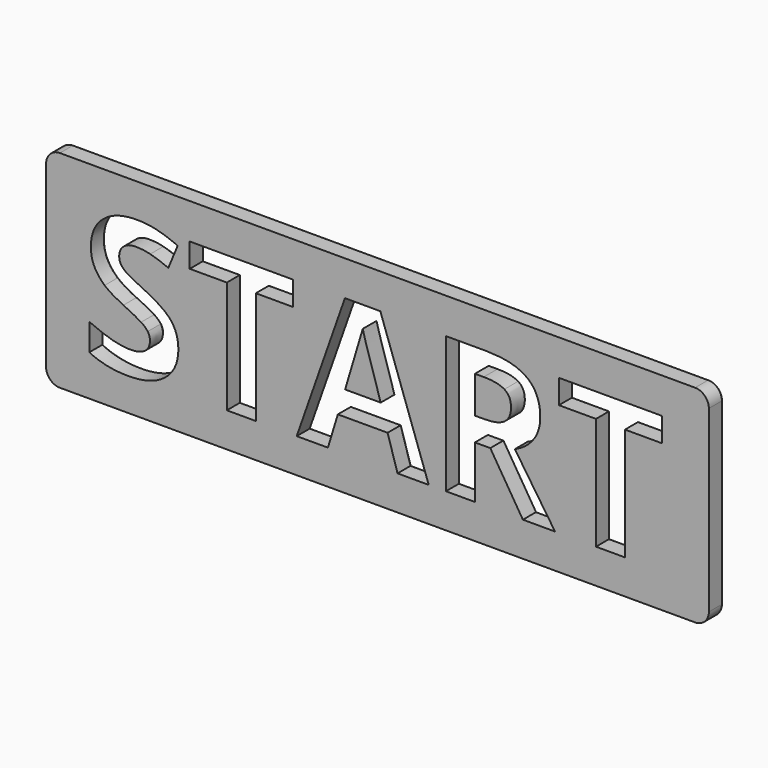
from build123d import *

# Parameters (mm, degrees)
F0_W     = 122.1989149306
F0_H     = 38.1
F1_DEPTH = 3.175
F2_R     = 2.54
F3_R     = 0.254


with BuildPart() as f1:
    # F0 (on Front) → F1 (new body)
    with BuildSketch(Plane.XZ):
        with Locations((54.7494574653, 12.7)):
            Rectangle(F0_W, F0_H)
        with BuildLine():
            add(Edge.make_bspline(
                [(16.7266276042, 11.1538411458), (18.0357638889, 9.4588541667), (18.0357638889, 6.994921875)],
                knots=[0, 0, 0, 1, 1, 1], degree=2))
            add(Edge.make_bspline(
                [(18.0357638889, 6.994921875), (18.0357638889, 3.5828993056), (15.5800998264, 1.6178168403)],
                knots=[0, 0, 0, 1, 1, 1], degree=2))
            add(Edge.make_bspline(
                [(15.5800998264, 1.6178168403), (13.1244357639, -0.347265625), (8.7532986111, -0.347265625)],
                knots=[0, 0, 0, 1, 1, 1], degree=2))
            add(Edge.make_bspline(
                [(8.7532986111, -0.347265625), (4.7184027778, -0.347265625), (1.6205729167, 1.1740885417)],
                knots=[0, 0, 0, 1, 1, 1], degree=2))
            Line((1.6205729167, 1.1740885417), (1.6205729167, 6.1350260417))
            add(Edge.make_bspline(
                [(1.6205729167, 6.1350260417), (4.1671875, 4.9940104167), (5.9338324653, 4.5309895833)],
                knots=[0, 0, 0, 1, 1, 1], degree=2))
            add(Edge.make_bspline(
                [(5.9338324653, 4.5309895833), (7.7004774306, 4.06796875), (9.1667100694, 4.06796875)],
                knots=[0, 0, 0, 1, 1, 1], degree=2))
            add(Edge.make_bspline(
                [(9.1667100694, 4.06796875), (10.9195746528, 4.06796875), (11.8593967014, 4.7376953125)],
                knots=[0, 0, 0, 1, 1, 1], degree=2))
            add(Edge.make_bspline(
                [(11.8593967014, 4.7376953125), (12.79921875, 5.407421875), (12.79921875, 6.7358506944)],
                knots=[0, 0, 0, 1, 1, 1], degree=2))
            add(Edge.make_bspline(
                [(12.79921875, 6.7358506944), (12.79921875, 7.4744791667), (12.3858072917, 8.0532552083)],
                knots=[0, 0, 0, 1, 1, 1], degree=2))
            add(Edge.make_bspline(
                [(12.3858072917, 8.0532552083), (11.9723958333, 8.63203125), (11.1703776042, 9.1639539931)],
                knots=[0, 0, 0, 1, 1, 1], degree=2))
            add(Edge.make_bspline(
                [(11.1703776042, 9.1639539931), (10.368359375, 9.6958767361), (7.9044270833, 10.8699652778)],
                knots=[0, 0, 0, 1, 1, 1], degree=2))
            add(Edge.make_bspline(
                [(7.9044270833, 10.8699652778), (5.6003472222, 11.955859375), (4.4455512153, 12.9535590278)],
                knots=[0, 0, 0, 1, 1, 1], degree=2))
            add(Edge.make_bspline(
                [(4.4455512153, 12.9535590278), (3.2907552083, 13.9512586806), (2.6017361111, 15.2796875)],
                knots=[0, 0, 0, 1, 1, 1], degree=2))
            add(Edge.make_bspline(
                [(2.6017361111, 15.2796875), (1.9127170139, 16.6081163194), (1.9127170139, 18.3775173611)],
                knots=[0, 0, 0, 1, 1, 1], degree=2))
            add(Edge.make_bspline(
                [(1.9127170139, 18.3775173611), (1.9127170139, 21.7233940972), (4.1782118056, 23.6333550347)],
                knots=[0, 0, 0, 1, 1, 1], degree=2))
            add(Edge.make_bspline(
                [(4.1782118056, 23.6333550347), (6.4437065972, 25.5433159722), (10.4400173611, 25.5433159722)],
                knots=[0, 0, 0, 1, 1, 1], degree=2))
            add(Edge.make_bspline(
                [(10.4400173611, 25.5433159722), (12.40234375, 25.5433159722), (14.1855251736, 25.0802951389)],
                knots=[0, 0, 0, 1, 1, 1], degree=2))
            add(Edge.make_bspline(
                [(14.1855251736, 25.0802951389), (15.9687065972, 24.6172743056), (17.9144965278, 23.7739149306)],
                knots=[0, 0, 0, 1, 1, 1], degree=2))
            Line((17.9144965278, 23.7739149306), (16.1947048611, 19.6177517361))
            add(Edge.make_bspline(
                [(16.1947048611, 19.6177517361), (14.1772569444, 20.4445746528), (12.8598524306, 20.7725477431)],
                knots=[0, 0, 0, 1, 1, 1], degree=2))
            add(Edge.make_bspline(
                [(12.8598524306, 20.7725477431), (11.5424479167, 21.1005208333), (10.269140625, 21.1005208333)],
                knots=[0, 0, 0, 1, 1, 1], degree=2))
            add(Edge.make_bspline(
                [(10.269140625, 21.1005208333), (8.7532986111, 21.1005208333), (7.9430121528, 20.3949652778)],
                knots=[0, 0, 0, 1, 1, 1], degree=2))
            add(Edge.make_bspline(
                [(7.9430121528, 20.3949652778), (7.1327256944, 19.6894097222), (7.1327256944, 18.55390625)],
                knots=[0, 0, 0, 1, 1, 1], degree=2))
            add(Edge.make_bspline(
                [(7.1327256944, 18.55390625), (7.1327256944, 17.8483506944), (7.4606987847, 17.3219401042)],
                knots=[0, 0, 0, 1, 1, 1], degree=2))
            add(Edge.make_bspline(
                [(7.4606987847, 17.3219401042), (7.788671875, 16.7955295139), (8.5024956597, 16.3049479167)],
                knots=[0, 0, 0, 1, 1, 1], degree=2))
            add(Edge.make_bspline(
                [(8.5024956597, 16.3049479167), (9.2163194444, 15.8143663194), (11.8842013889, 14.5410590278)],
                knots=[0, 0, 0, 1, 1, 1], degree=2))
            add(Edge.make_bspline(
                [(11.8842013889, 14.5410590278), (15.4174913194, 12.848828125), (16.7266276042, 11.1538411458)],
                knots=[0, 0, 0, 1, 1, 1], degree=2))
        make_face(mode=Mode.SUBTRACT)
        Polygon((32.3177517361, 20.7422309028), (32.3177517361, 0), (26.9764756944, 0), (26.9764756944, 20.7422309028), (20.1358940972, 20.7422309028), (20.1358940972, 25.1850260417), (39.1528211806, 25.1850260417), (39.1528211806, 20.7422309028), align=None, mode=Mode.SUBTRACT)
        Polygon((64.2000434028, 0), (58.4453559028, 0), (56.6208333333, 5.9972222222), (47.4375868056, 5.9972222222), (45.6130642361, 0), (39.8583767361, 0), (48.7494791667, 25.2897569444), (55.2758680556, 25.2897569444), align=None, mode=Mode.SUBTRACT)
        with BuildLine():
            Line((75.5495659722, 9.6628038194), (72.7108072917, 9.6628038194))
            Line((72.7108072917, 9.6628038194), (72.7108072917, 0))
            Line((72.7108072917, 0), (67.36953125, 0))
            Line((67.36953125, 0), (67.36953125, 25.1850260417))
            Line((67.36953125, 25.1850260417), (74.7062065972, 25.1850260417))
            add(Edge.make_bspline(
                [(74.7062065972, 25.1850260417), (79.8435329861, 25.1850260417), (82.3047092014, 23.31640625)],
                knots=[0, 0, 0, 1, 1, 1], degree=2))
            add(Edge.make_bspline(
                [(82.3047092014, 23.31640625), (84.7658854167, 21.4477864583), (84.7658854167, 17.6388888889)],
                knots=[0, 0, 0, 1, 1, 1], degree=2))
            add(Edge.make_bspline(
                [(84.7658854167, 17.6388888889), (84.7658854167, 15.4174913194), (83.5449435764, 13.6866753472)],
                knots=[0, 0, 0, 1, 1, 1], degree=2))
            add(Edge.make_bspline(
                [(83.5449435764, 13.6866753472), (82.3240017361, 11.955859375), (80.0805555556, 10.9746961806)],
                knots=[0, 0, 0, 1, 1, 1], degree=2))
            add(Edge.make_bspline(
                [(80.0805555556, 10.9746961806), (85.7690972222, 2.48046875), (87.4888888889, 0)],
                knots=[0, 0, 0, 1, 1, 1], degree=2))
            Line((87.4888888889, 0), (81.5633246528, 0))
            Line((81.5633246528, 0), (75.5495659722, 9.6628038194))
        make_face(mode=Mode.SUBTRACT)
        Polygon((100.3763020833, 20.7422309028), (100.3763020833, 0), (95.0350260417, 0), (95.0350260417, 20.7422309028), (88.1944444444, 20.7422309028), (88.1944444444, 25.1850260417), (107.2113715278, 25.1850260417), (107.2113715278, 20.7422309028), align=None, mode=Mode.SUBTRACT)
    extrude(amount=F1_DEPTH)

    # F2
    f2_edges = [f1.edges().sort_by_distance(p)[0] for p in [
        (-6.35, -1.5875, -6.35),
        (-6.35, -1.5875, 31.75),
        (115.848915, -1.5875, -6.35),
        (115.848915, -1.5875, 31.75),
    ]]
    fillet(f2_edges, radius=F2_R)

    # F3
    f3_edges = [f1.edges().sort_by_distance(p)[0] for p in [
        (54.749457, 0, 31.75),
        (115.104966, 0, 31.006051),
        (-5.606051, 0, 31.006051),
        (115.848915, 0, 12.7),
        (-6.35, 0, 12.7),
        (115.104966, 0, -5.606051),
        (-5.606051, 0, -5.606051),
        (54.749457, 0, -6.35),
        (17.732825, 0, 9.187508),
        (17.450639, 0, 4.008638),
        (12.341387, 0, 0.061322),
        (5.097382, 0, 0.002912),
        (1.620573, 0, 3.654557),
        (3.746225, 0, 5.248589),
        (7.535945, 0, 4.196852),
        (10.56702, 0, 4.200862),
        (12.58346, 0, 5.614068),
        (12.697954, 0, 7.427825),
        (11.828227, 0, 8.662696),
        (9.559736, 0, 10.058857),
        (6.108329, 0, 11.803246),
        (3.411842, 0, 14.02809),
        (2.070301, 0, 16.785996),
        (2.44012, 0, 21.271954),
        (7.132146, 0, 25.139853),
        (12.327657, 0, 25.431226),
        (16.075107, 0, 24.499056),
        (17.054601, 0, 21.695833),
        (14.546599, 0, 20.251719),
        (11.574458, 0, 21.01585),
        (9.039214, 0, 20.955371),
        (7.328909, 0, 19.567265),
        (7.209225, 0, 17.914183),
        (7.929957, 0, 16.761471),
        (10.170242, 0, 15.379812),
        (14.488954, 0, 13.100075),
        (32.317752, 0, 10.371115),
        (29.647114, 0, 0),
        (26.976476, 0, 10.371115),
        (23.556185, 0, 20.742231),
        (20.135894, 0, 22.963628),
        (29.644358, 0, 25.185026),
        (39.152821, 0, 22.963628),
        (35.735286, 0, 20.742231),
        (61.3227, 0, 0),
        (57.533095, 0, 2.998611),
        (52.02921, 0, 5.997222),
        (46.525326, 0, 2.998611),
        (42.73572, 0, 0),
        (44.303928, 0, 12.644878),
        (52.012674, 0, 25.289757),
        (59.737956, 0, 12.644878),
        (74.130187, 0, 9.662804),
        (72.710807, 0, 4.831402),
        (70.040169, 0, 0),
        (67.369531, 0, 12.592513),
        (71.037869, 0, 25.185026),
        (78.662357, 0, 24.832852),
        (84.22336, 0, 20.787767),
        (84.468402, 0, 15.565413),
        (82.001826, 0, 12.091742),
        (83.770154, 0, 5.477491),
        (84.526107, 0, 0),
        (78.556445, 0, 4.831402),
        (100.376302, 0, 10.371115),
        (97.705664, 0, 0),
        (95.035026, 0, 10.371115),
        (91.614735, 0, 20.742231),
        (88.194444, 0, 22.963628),
        (97.702908, 0, 25.185026),
        (107.211372, 0, 22.963628),
        (103.793837, 0, 20.742231),
    ]]
    fillet(f3_edges, radius=F3_R)


with BuildPart() as f1b:
    # F0 (on Front) → F1, piece 2 (new body)
    with BuildSketch(Plane.XZ):
        with BuildLine():
            Line((72.7108072917, 20.8083767361), (72.7108072917, 14.0063802083))
            Line((72.7108072917, 14.0063802083), (74.4305989583, 14.0063802083))
            add(Edge.make_bspline(
                [(74.4305989583, 14.0063802083), (76.9661892361, 14.0063802083), (78.1705946181, 14.8497395833)],
                knots=[0, 0, 0, 1, 1, 1], degree=2))
            add(Edge.make_bspline(
                [(78.1705946181, 14.8497395833), (79.375, 15.6930989583), (79.375, 17.5010850694)],
                knots=[0, 0, 0, 1, 1, 1], degree=2))
            add(Edge.make_bspline(
                [(79.375, 17.5010850694), (79.375, 19.2925347222), (78.1430338542, 20.0504557292)],
                knots=[0, 0, 0, 1, 1, 1], degree=2))
            add(Edge.make_bspline(
                [(78.1430338542, 20.0504557292), (76.9110677083, 20.8083767361), (74.3313802083, 20.8083767361)],
                knots=[0, 0, 0, 1, 1, 1], degree=2))
            Line((74.3313802083, 20.8083767361), (72.7108072917, 20.8083767361))
        make_face()
    extrude(amount=F1_DEPTH)


with BuildPart() as f1c:
    # F0 (on Front) → F1, piece 3 (new body)
    with BuildSketch(Plane.XZ):
        with BuildLine():
            Line((48.7825520833, 10.4730902778), (55.3420138889, 10.4730902778))
            add(Edge.make_bspline(
                [(55.3420138889, 10.4730902778), (52.8119357639, 18.6200520833), (52.4922309028, 19.6894097222)],
                knots=[0, 0, 0, 1, 1, 1], degree=2))
            add(Edge.make_bspline(
                [(52.4922309028, 19.6894097222), (52.1725260417, 20.7587673611), (52.0347222222, 21.3761284722)],
                knots=[0, 0, 0, 1, 1, 1], degree=2))
            add(Edge.make_bspline(
                [(52.0347222222, 21.3761284722), (51.4669704861, 19.1712673611), (48.7825520833, 10.4730902778)],
                knots=[0, 0, 0, 1, 1, 1], degree=2))
        make_face()
    extrude(amount=F1_DEPTH)


solid = Compound([f1.part, f1b.part, f1c.part])
